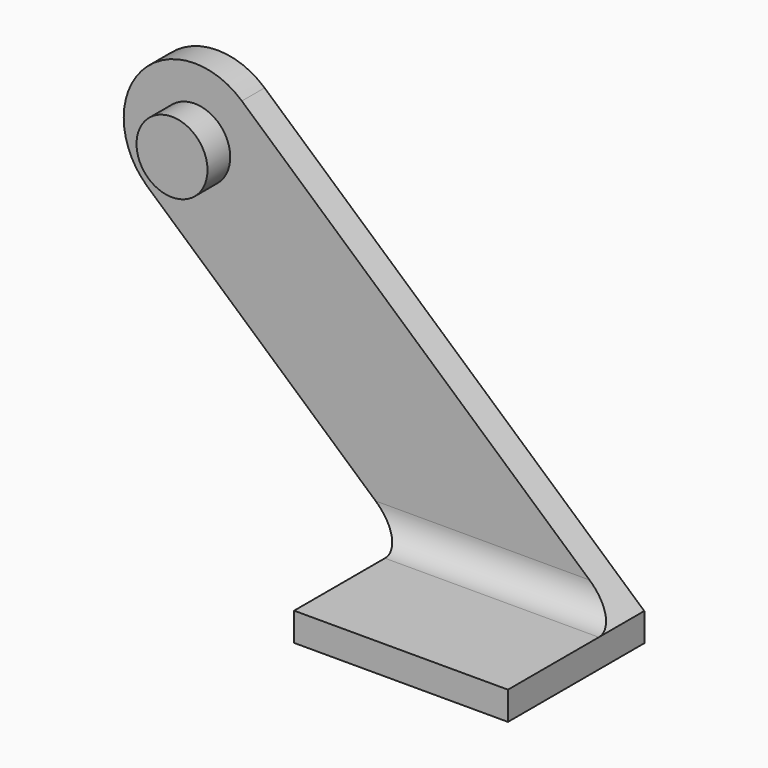
from build123d import *

# Parameters (mm, degrees)
F0_R          = 2.5
F1_DEPTH      = 2
F0_W          = 15.064
F0_H          = 2
F2_DEPTH      = 10
F2_DEPTH_BACK = 2
F3_DEPTH      = 2
F3_DEPTH_BACK = 2
F4_R          = 2


# Not quite as in the source:
# - ends of sketch curves that miss each other by under 0.0002 mm in the source are joined


with BuildPart() as f1:
    # F0 (on Front) → F1 (new body)
    with BuildSketch(Plane.XZ):
        with BuildLine():
            Line((30.0639452948, -20), (3.3191835885, 3.7393876913))
            ThreePointArc((3.3191835885, 3.7393876913), (-3.7393876913, 3.3191835885), (-3.3191835885, -3.7393876913))
            Line((-3.3191835885, -3.7393876913), (15, -20))
            Line((15, -20), (30.0639452948, -20))
        make_face()
        Circle(F0_R, mode=Mode.SUBTRACT)
    extrude(amount=-F1_DEPTH)

    # F0 (on Front) → F2 (join, two sides)
    with BuildSketch(Plane.XZ) as f2_sk:
        with Locations((22.532, -21)):
            Rectangle(F0_W, F0_H)
    extrude(amount=F2_DEPTH)
    extrude(f2_sk.sketch, amount=-F2_DEPTH_BACK)

    # F0 (on Front) → F3 (join, two sides)
    with BuildSketch(Plane.XZ) as f3_sk:
        Circle(F0_R)
    extrude(amount=F3_DEPTH)
    extrude(f3_sk.sketch, amount=-F3_DEPTH_BACK)

    # F4
    f4_edges = [f1.edges().sort_by_distance(p)[0] for p in [
        (22.531973, 0, -20),
    ]]
    fillet(f4_edges, radius=F4_R)


solid = f1.part
